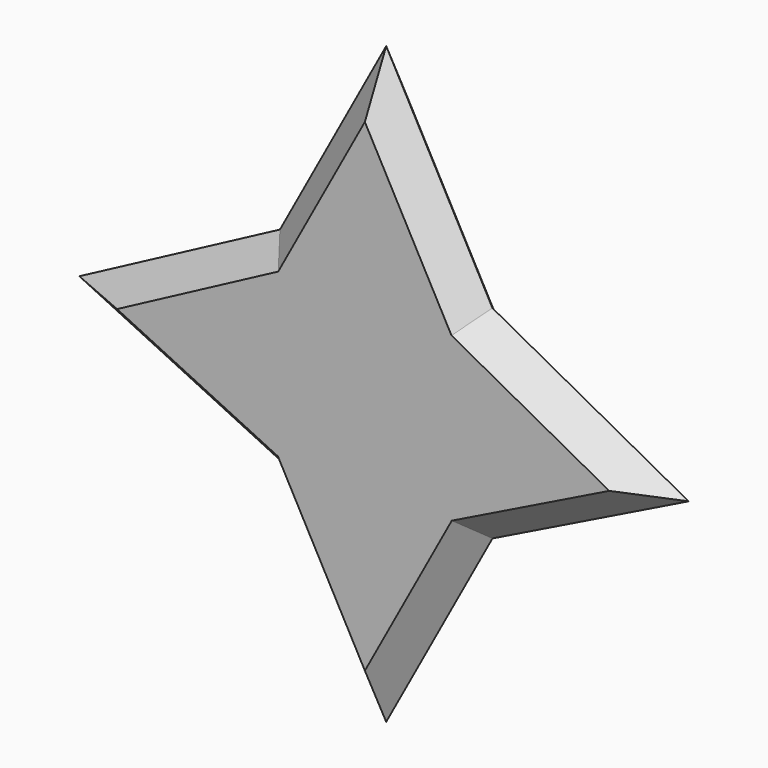
from build123d import *

# Parameters (mm, degrees)
F1_DEPTH = 10.16
F2_SIZE  = 5.07999


# Not quite as in the source:
# - a fillet or chamfer is up to 0.001 mm smaller than in the source, because OpenCascade refuses the exact size


with BuildPart() as f1:
    # F0 (on Front) → F1 (new body)
    with BuildSketch(Plane.XZ):
        Polygon((20.2520862222, 38.6501066387), (0, 76.0166272521), (-20.2520843595, 38.6501066387), (-58.4743283689, 18.3879856241), (-20.2520843595, 0), (0, -37.3665240501), (20.2520862222, 0), (57.6371251704, 18.3879856241), align=None)
    extrude(amount=F1_DEPTH)

    # F2 (size 5.08 in the source; OpenCascade refuses exactly that, so slightly less here)
    f2_edges = [f1.edges().sort_by_distance(p)[0] for p in [
        (-39.363206, -10.16, 28.519046),
        (-10.126042, -10.16, 57.333367),
        (10.126043, -10.16, 57.333367),
        (38.944606, -10.16, 28.519046),
        (38.944606, -10.16, 9.193993),
        (10.126043, -10.16, -18.683262),
        (-10.126042, -10.16, -18.683262),
        (-39.363206, -10.16, 9.193993),
        (10.126043, 0, 57.333367),
        (-10.126042, 0, 57.333367),
        (-39.363206, 0, 28.519046),
        (-39.363206, 0, 9.193993),
        (-10.126042, 0, -18.683262),
        (10.126043, 0, -18.683262),
        (38.944606, 0, 9.193993),
        (38.944606, 0, 28.519046),
    ]]
    chamfer(f2_edges, length=F2_SIZE)


solid = f1.part
